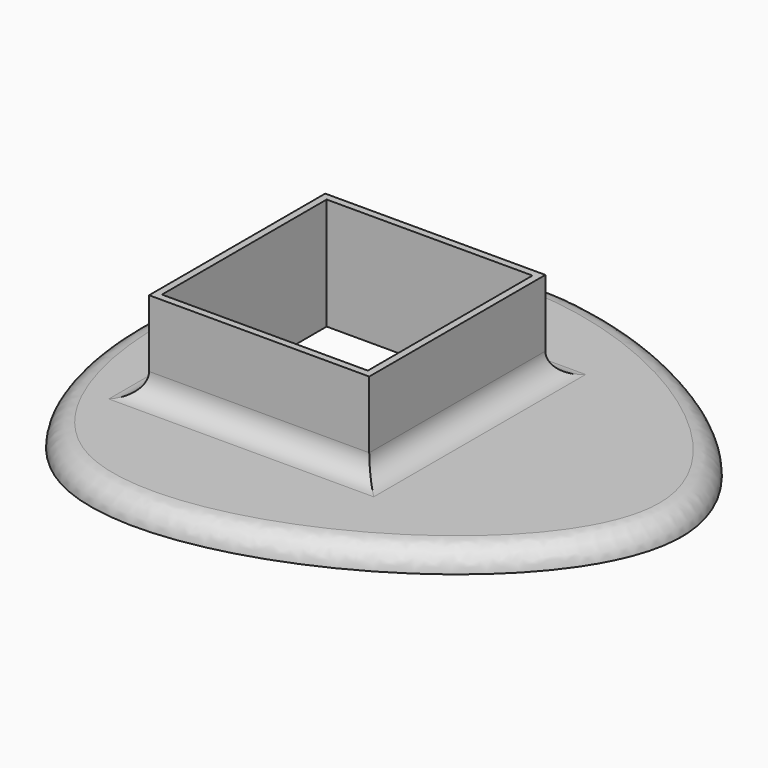
from build123d import *

# Parameters (mm, degrees)
F1_DEPTH = 5
F2_DEPTH = 25
F3_R     = 4.99999


# Not quite as in the source:
# - a fillet or chamfer is up to 0.001 mm smaller than in the source, because OpenCascade refuses the exact size


with BuildPart() as f1:
    # F0 (on Top) → F1 (new body)
    with BuildSketch(Plane.XY):
        with BuildLine():
            add(Edge.make_bspline(
                [(0, 47.6761966849), (31.7996343084, 66.3650460849), (162.4107710873, 1.1493064278), (-0.5654891103, -87.7590913423), (-23.5407682827, -21.5589349291), (-22.8451150266, 0)],
                knots=[0, 0, 0, 0, 0.3365827736, 0.6764560587, 0.845419572, 0.845419572, 0.845419572, 0.845419572], degree=3))
            add(Edge.make_bspline(
                [(-22.8451150266, 0), (-22.2086795266, 19.7237221407), (-14.6044345316, 39.0930766752), (0, 47.6761966849)],
                knots=[0.845419572, 0.845419572, 0.845419572, 0.845419572, 1, 1, 1, 1], degree=3))
        make_face()
        Polygon((-2.4451150266, -24.6), (-2.4451150266, 0), (-2.4451150266, 24.6), (46.7548849734, 24.6), (46.7548849734, -24.6), align=None, mode=Mode.SUBTRACT)
    extrude(amount=F1_DEPTH)

    # F0 (on Top) → F2 (join)
    with BuildSketch(Plane.XY):
        Polygon((-2.4451150266, 24.6), (-2.4451150266, 0), (-2.4451150266, -24.6), (46.7548849734, -24.6), (46.7548849734, 24.6), align=None)
        Polygon((-0.8451150266, -23), (-0.8451150266, 0), (-0.8451150266, 23), (45.1548849734, 23), (45.1548849734, -23), align=None, mode=Mode.SUBTRACT)
    extrude(amount=F2_DEPTH)

    # F3 (radius 5 in the source; OpenCascade refuses exactly that, so slightly less here)
    f3_edges = [f1.edges().sort_by_distance(p)[0] for p in [
        (46.754885, 0, 5),
        (22.154885, -24.6, 5),
        (-2.445115, 0, 5),
        (22.154885, 24.6, 5),
        (84.577965, -27.452992, 5),
    ]]
    fillet(f3_edges, radius=F3_R)


solid = f1.part
